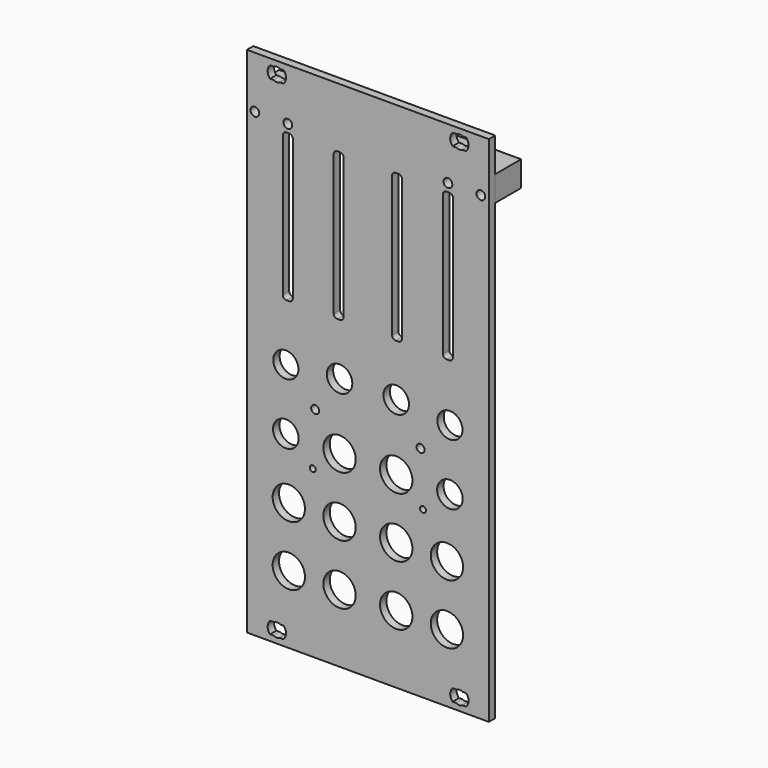
from build123d import *

# Parameters (mm, degrees)
F0_R     = 4.05
F0_R_2   = 3.200001
F0_R_3   = 3.15
F0_R_4   = 0.75
F0_R_5   = 1
F0_R_6   = 1.1
F1_DEPTH = 2
F2_W     = 60.600001
F2_H     = 6.35
F2_R     = 1.1
F3_DEPTH = 8.1
F4_R     = 1.1
F5_DEPTH = 25


# Not quite as in the source:
# - ends of sketch curves that miss each other by under 0.0002 mm in the source are joined


with BuildPart() as f1:
    # F0 (on Front) → F1 (new body)
    with BuildSketch(Plane.XZ):
        Polygon((-30.3, -61.250013), (-30.3, -64.250012), (30.300001, -64.250012), (30.300001, 64.250011), (-30.3, 64.250011), align=None)
        with BuildLine():
            ThreePointArc((-23.600001, -59.750013), (-22.7999995588, -59.550011), (-21.9999982215, -59.7500134152))
            Line((-21.9999982215, -59.7500134152), (-21.100001, -59.750013))
            ThreePointArc((-21.100001, -59.750013), (-20.5, -61.2500126379), (-21.1000001998, -62.7500108097))
            Line((-21.1000001998, -62.7500108097), (-21.999999, -62.750012))
            ThreePointArc((-21.999999, -62.750012), (-22.7999995588, -62.950014), (-23.600001, -62.750012))
            Line((-23.600001, -62.750012), (-24.499999, -62.750012))
            ThreePointArc((-24.499999, -62.750012), (-25.1, -61.2500126379), (-24.4999988252, -59.7500141665))
            Line((-24.4999988252, -59.7500141665), (-23.600001, -59.750013))
        make_face(mode=Mode.SUBTRACT)
        with Locations((-19.800001, -47.249931)):
            Circle(F0_R, mode=Mode.SUBTRACT)
        with Locations((-19.800052, -32.249984)):
            Circle(F0_R, mode=Mode.SUBTRACT)
        with Locations((-7.100001, -47.249931)):
            Circle(F0_R, mode=Mode.SUBTRACT)
        with Locations((-7.100052, -32.249984)):
            Circle(F0_R, mode=Mode.SUBTRACT)
        with Locations((-20.549999, -17.249989)):
            Circle(F0_R_2, mode=Mode.SUBTRACT)
        with Locations((-20.549999, -1.999989)):
            Circle(F0_R_3, mode=Mode.SUBTRACT)
        with Locations((-13.8, -22.749991)):
            Circle(F0_R_4, mode=Mode.SUBTRACT)
        with Locations((-7.100052, -17.249986)):
            Circle(F0_R, mode=Mode.SUBTRACT)
        with Locations((-13.200001, -9.499989)):
            Circle(F0_R_5, mode=Mode.SUBTRACT)
        with Locations((-7.100001, -0.749989)):
            Circle(F0_R_2, mode=Mode.SUBTRACT)
        with Locations((7.099976, -47.249957)):
            Circle(F0_R, mode=Mode.SUBTRACT)
        with Locations((7.09995, -32.249928)):
            Circle(F0_R, mode=Mode.SUBTRACT)
        with BuildLine():
            ThreePointArc((22.119986, -59.750023), (22.9199874412, -59.550021), (23.7199887785, -59.7500234152))
            Line((23.7199887785, -59.7500234152), (24.619987, -59.750023))
            ThreePointArc((24.619987, -59.750023), (25.219987, -61.250023), (24.6199863008, -62.7500213341))
            Line((24.6199863008, -62.7500213341), (23.719988, -62.750022))
            ThreePointArc((23.719988, -62.750022), (22.9199874412, -62.950024), (22.119986, -62.750022))
            Line((22.119986, -62.750022), (21.219988, -62.750022))
            ThreePointArc((21.219988, -62.750022), (20.619987, -61.250023), (21.2199901249, -59.7500221189))
            Line((21.2199901249, -59.7500221189), (22.119986, -59.750023))
        make_face(mode=Mode.SUBTRACT)
        with Locations((19.799976, -47.249957)):
            Circle(F0_R, mode=Mode.SUBTRACT)
        with Locations((19.79995, -32.249928)):
            Circle(F0_R, mode=Mode.SUBTRACT)
        with Locations((7.099925, -17.249928)):
            Circle(F0_R, mode=Mode.SUBTRACT)
        with Locations((13.799975, -22.749991)):
            Circle(F0_R_4, mode=Mode.SUBTRACT)
        with Locations((7.100052, -0.749989)):
            Circle(F0_R_2, mode=Mode.SUBTRACT)
        with Locations((13.199999, -9.499989)):
            Circle(F0_R_5, mode=Mode.SUBTRACT)
        with Locations((20.549974, -17.249989)):
            Circle(F0_R_2, mode=Mode.SUBTRACT)
        with Locations((20.549974, -1.999989)):
            Circle(F0_R_3, mode=Mode.SUBTRACT)
        with BuildLine():
            Line((-21.3, 13.150011), (-21.3, 30.750012))
            Line((-21.3, 30.750012), (-21.3, 48.350012))
            ThreePointArc((-21.3, 48.350012), (-21.0363968102, 48.9864088102), (-20.4, 49.250013))
            Line((-20.4, 49.250013), (-19.700001, 49.250013))
            ThreePointArc((-19.700001, 49.250013), (-19.0636041898, 48.9864088102), (-18.8, 48.350012))
            Line((-18.8, 48.350012), (-18.8, 30.750012))
            Line((-18.8, 30.750012), (-18.8, 13.150011))
            ThreePointArc((-18.8, 13.150011), (-19.0636041898, 12.5136141898), (-19.700001, 12.25001))
            Line((-19.700001, 12.25001), (-20.4, 12.250011))
            ThreePointArc((-20.4, 12.250011), (-21.0363968102, 12.5136141898), (-21.3, 13.150011))
        make_face(mode=Mode.SUBTRACT)
        with BuildLine():
            Line((-8.55, 13.150011), (-8.55, 30.750012))
            Line((-8.55, 30.750012), (-8.55, 48.350012))
            ThreePointArc((-8.55, 48.350012), (-8.2863968102, 48.9864088102), (-7.65, 49.250013))
            Line((-7.65, 49.250013), (-6.950001, 49.250013))
            ThreePointArc((-6.950001, 49.250013), (-6.3136041898, 48.9864088102), (-6.05, 48.350012))
            Line((-6.05, 48.350012), (-6.05, 30.750012))
            Line((-6.05, 30.750012), (-6.05, 13.150011))
            ThreePointArc((-6.05, 13.150011), (-6.3136041898, 12.5136141898), (-6.950001, 12.25001))
            Line((-6.950001, 12.25001), (-7.65, 12.250011))
            ThreePointArc((-7.65, 12.250011), (-8.2863968102, 12.5136141898), (-8.55, 13.150011))
        make_face(mode=Mode.SUBTRACT)
        with BuildLine():
            ThreePointArc((-23.600014, 62.750001), (-22.8000125588, 62.950003), (-22.0000112215, 62.7500005848))
            Line((-22.0000112215, 62.7500005848), (-21.100013, 62.750001))
            ThreePointArc((-21.100013, 62.750001), (-20.500013, 61.2500013621), (-21.1000131998, 59.7500031903))
            Line((-21.1000131998, 59.7500031903), (-22.000012, 59.750002))
            ThreePointArc((-22.000012, 59.750002), (-22.8000125588, 59.55), (-23.600014, 59.750002))
            Line((-23.600014, 59.750002), (-24.500012, 59.750002))
            ThreePointArc((-24.500012, 59.750002), (-25.100013, 61.2500013621), (-24.5000093757, 62.7500024055))
            Line((-24.5000093757, 62.7500024055), (-23.600014, 62.750001))
        make_face(mode=Mode.SUBTRACT)
        with Locations((-20.049998, 51.250011)):
            Circle(F0_R_6, mode=Mode.SUBTRACT)
        with BuildLine():
            Line((6.050001, 13.150011), (6.050001, 30.750012))
            Line((6.050001, 30.750012), (6.050001, 48.350012))
            ThreePointArc((6.050001, 48.350012), (6.3136051898, 48.9864088102), (6.950002, 49.250013))
            Line((6.950002, 49.250013), (7.65, 49.250013))
            ThreePointArc((7.65, 49.250013), (8.2863968102, 48.9864088102), (8.550001, 48.350012))
            Line((8.550001, 48.350012), (8.550001, 30.750012))
            Line((8.550001, 30.750012), (8.550001, 13.150011))
            ThreePointArc((8.550001, 13.150011), (8.2863968102, 12.5136141898), (7.65, 12.25001))
            Line((7.65, 12.25001), (6.950002, 12.250011))
            ThreePointArc((6.950002, 12.250011), (6.3136051898, 12.5136141898), (6.050001, 13.150011))
        make_face(mode=Mode.SUBTRACT)
        with BuildLine():
            Line((18.800001, 13.150009), (18.800001, 30.750009))
            Line((18.800001, 30.750009), (18.800001, 48.35001))
            ThreePointArc((18.800001, 48.35001), (19.0636041898, 48.9864068102), (19.700001, 49.250011))
            Line((19.700001, 49.250011), (20.4, 49.25001))
            ThreePointArc((20.4, 49.25001), (21.0363968102, 48.9864068102), (21.300001, 48.35001))
            Line((21.300001, 48.35001), (21.300001, 30.750009))
            Line((21.300001, 30.750009), (21.300001, 13.150009))
            ThreePointArc((21.300001, 13.150009), (21.0363968102, 12.5136121898), (20.4, 12.250008))
            Line((20.4, 12.250008), (19.700001, 12.250008))
            ThreePointArc((19.700001, 12.250008), (19.0636041898, 12.5136121898), (18.800001, 13.150009))
        make_face(mode=Mode.SUBTRACT)
        with Locations((20.050001, 51.250009)):
            Circle(F0_R_6, mode=Mode.SUBTRACT)
        with BuildLine():
            Line((22.119986, 59.750002), (21.219988, 59.750002))
            ThreePointArc((21.219988, 59.750002), (20.619987, 61.2500013621), (21.2199906243, 62.7500024055))
            Line((21.2199906243, 62.7500024055), (22.119986, 62.750001))
            ThreePointArc((22.119986, 62.750001), (22.9199874412, 62.950003), (23.7199887785, 62.7500005848))
            Line((23.7199887785, 62.7500005848), (24.619987, 62.750001))
            ThreePointArc((24.619987, 62.750001), (25.219987, 61.2500013621), (24.6199868002, 59.7500031903))
            Line((24.6199868002, 59.7500031903), (23.719988, 59.750002))
            ThreePointArc((23.719988, 59.750002), (22.9199874412, 59.55), (22.119986, 59.750002))
        make_face(mode=Mode.SUBTRACT)
    extrude(amount=F1_DEPTH)

    # F4 (on face) → F5 (cut)
    with BuildSketch(Plane(origin=(0, 0, 0), x_dir=(-1, 0, 0), z_dir=(0, 1, 0))):
        with Locations((-28.300001, 51.250009)):
            Circle(F4_R)
        with Locations((28.3, 51.250009)):
            Circle(F4_R)
    extrude(amount=-F5_DEPTH, mode=Mode.SUBTRACT)


with BuildPart() as f3:
    # F2 (on face) → F3 (new body)
    with BuildSketch(Plane(origin=(0, 0, 0), x_dir=(-1, 0, 0), z_dir=(0, 1, 0))):
        with Locations((-5e-07, 52.5382029457)):
            Rectangle(F2_W, F2_H)
        with Locations((-28.300001, 51.250009)):
            Circle(F2_R, mode=Mode.SUBTRACT)
        with Locations((-20.050001, 51.250009)):
            Circle(F2_R, mode=Mode.SUBTRACT)
        with Locations((20.049998, 51.250011)):
            Circle(F2_R, mode=Mode.SUBTRACT)
        with Locations((28.3, 51.250009)):
            Circle(F2_R, mode=Mode.SUBTRACT)
    extrude(amount=F3_DEPTH)


solid = Compound([f1.part, f3.part])
